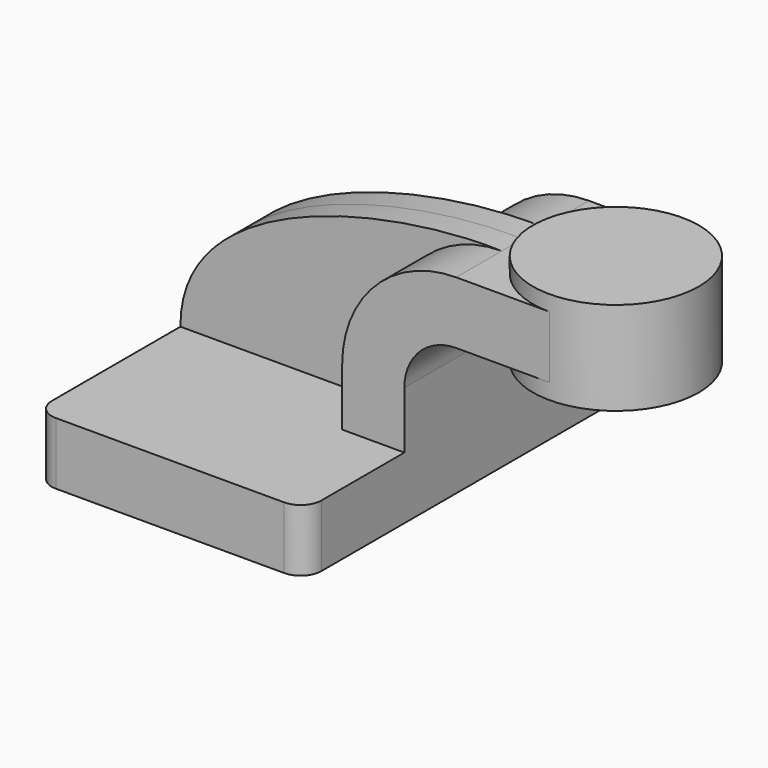
from build123d import *

# Parameters (mm, degrees)
F1_DEPTH = 63.5
F2_DEPTH = 25.4
F3_DEPTH = 7.9375
F5_R     = 6.35


with BuildPart() as f1:
    # F0 (on Front) → F1 (new body, symmetric)
    with BuildSketch(Plane.XZ):
        Polygon((22.225, 9.525), (-41.275, 9.525), (-41.275, -9.525), (41.275, -9.525), (41.275, 9.525), align=None)
    extrude(amount=F1_DEPTH, both=True)

    # F0 (on Front) → F2 (join, symmetric)
    with BuildSketch(Plane.XZ):
        with BuildLine():
            Line((22.225, 27.0002), (22.225, 9.525))
            Line((22.225, 9.525), (41.275, 9.525))
            Line((41.275, 9.525), (41.275, 27.0002))
            ThreePointArc((41.275, 27.0002), (45.9246798487, 38.2255201513), (57.15, 42.8752))
            Line((57.15, 42.8752), (60.325, 42.8752))
            Line((60.325, 42.8752), (60.325, 61.9252))
            Line((60.325, 61.9252), (57.15, 61.9252))
            ThreePointArc((57.15, 61.9252), (32.4542956671, 51.6959043329), (22.225, 27.0002))
        make_face()
        Polygon((85.725, 61.9252), (60.325, 61.9252), (60.325, 42.8752), (85.725, 42.8752), (85.725, 52.3875), align=None)
    extrude(amount=F2_DEPTH, both=True)

    # F0 (on Front) → F3 (join, symmetric)
    with BuildSketch(Plane.XZ):
        with BuildLine():
            add(Edge.make_bspline(
                [(-41.275, 9.525), (-41.5751747787, 48.5781729221), (22.9490175843, 63.0326196551), (57.15, 61.9252)],
                knots=[0, 0, 0, 0, 111.5045361635, 111.5045361635, 111.5045361635, 111.5045361635], degree=3))
            Line((-41.275, 9.525), (22.225, 9.525))
            Line((22.225, 9.525), (22.225, 27.0002))
            ThreePointArc((22.225, 27.0002), (32.4542956671, 51.6959043329), (57.15, 61.9252))
        make_face()
    extrude(amount=F3_DEPTH, both=True)

    # F0 (on Front) → F4 (revolve)
    with BuildSketch(Plane.XZ):
        Polygon((85.725, 66.675), (85.725, 61.9252), (85.725, 52.3875), (85.725, 42.8752), (85.725, 38.1), (111.125, 38.1), (111.125, 66.675), align=None)
    revolve(axis=Axis((85.725, 0, 21.2952332962), (0, 0, -1)))

    # F5
    f5_edges = [f1.edges().sort_by_distance(p)[0] for p in [
        (41.275, -63.5, 0),
        (-41.275, -63.5, 0),
        (-41.275, 63.5, 0),
        (41.275, 63.5, 0),
    ]]
    fillet(f5_edges, radius=F5_R)


solid = f1.part
